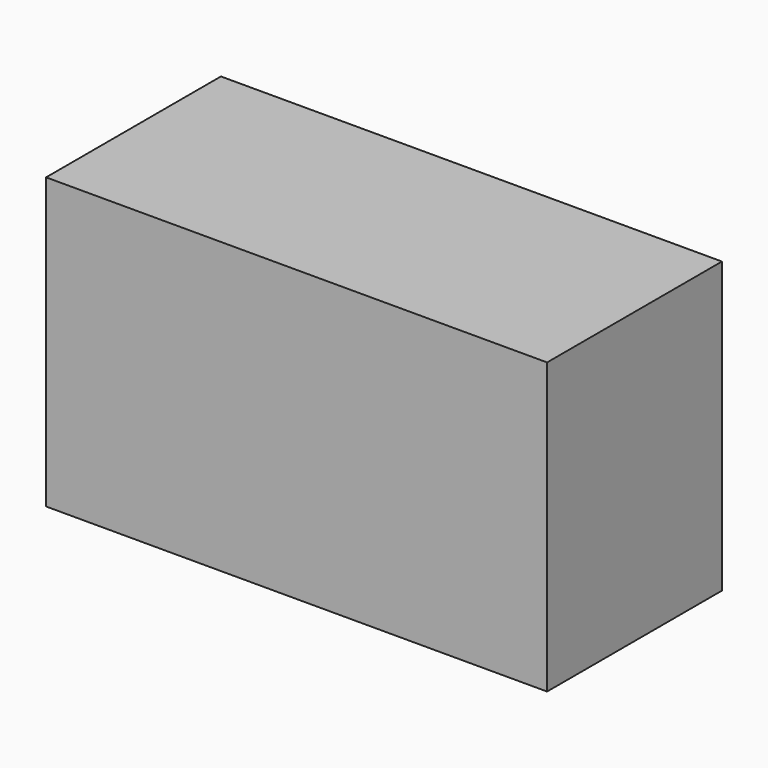
from build123d import *

# Parameters (mm, degrees)
F0_W     = 219.5894941688
F0_H     = 95.7783982158
F1_DEPTH = 127


# Not quite as in the source:
# - the program builds the solid bodies; features that only make, move or delete a surface that nothing else refers to are left out


with BuildPart() as f1:
    # F0 (on Top) → F1 (new body)
    with BuildSketch(Plane.XY):
        with Locations((34.0188480914, 15.3303854167)):
            Rectangle(F0_W, F0_H)
    extrude(amount=F1_DEPTH)


solid = f1.part
